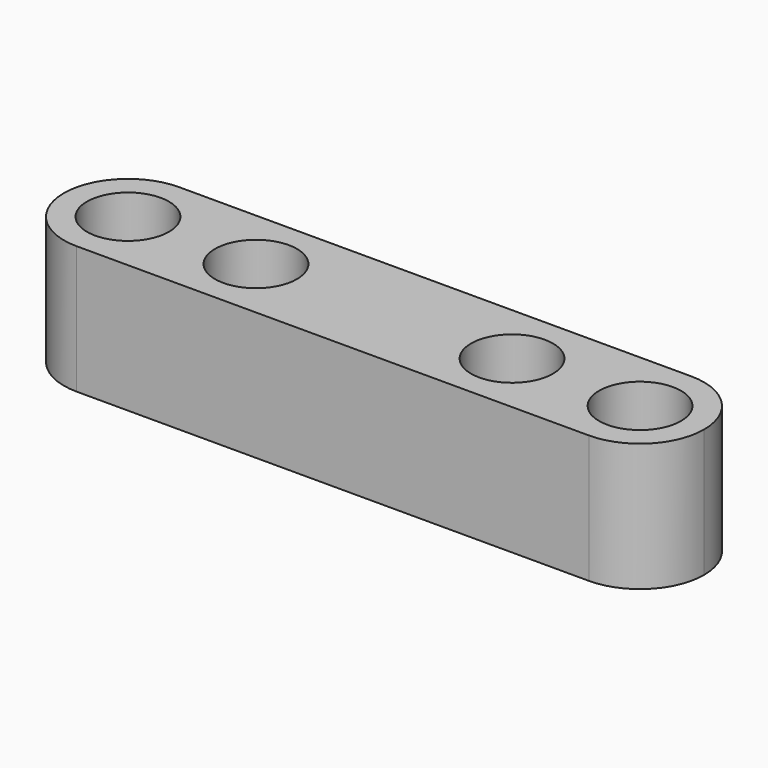
from build123d import *

# Parameters (mm, degrees)
F0_W     = 39.6875
F0_H     = 7.9375
F0_R     = 2.54
F1_DEPTH = 7.9375
F2_R     = 3.96874


# Not quite as in the source:
# - a fillet or chamfer is up to 0.001 mm smaller than in the source, because OpenCascade refuses the exact size


with BuildPart() as f1:
    # F0 (on Top) → F1 (new body)
    with BuildSketch(Plane.XY):
        with Locations((19.84375, -3.96875)):
            Rectangle(F0_W, F0_H)
        with Locations((3.96875, -3.96875)):
            Circle(F0_R, mode=Mode.SUBTRACT)
        with Locations((11.90625, -3.96875)):
            Circle(F0_R, mode=Mode.SUBTRACT)
        with Locations((27.78125, -3.96875)):
            Circle(F0_R, mode=Mode.SUBTRACT)
        with Locations((35.71875, -3.96875)):
            Circle(F0_R, mode=Mode.SUBTRACT)
    extrude(amount=F1_DEPTH)

    # F2 (radius 3.96875 in the source; OpenCascade refuses exactly that, so slightly less here)
    f2_edges = [f1.edges().sort_by_distance(p)[0] for p in [
        (0, 0, 3.96875),
        (0, -7.9375, 3.96875),
        (39.6875, -7.9375, 3.96875),
        (39.6875, 0, 3.96875),
    ]]
    fillet(f2_edges, radius=F2_R)


solid = f1.part
